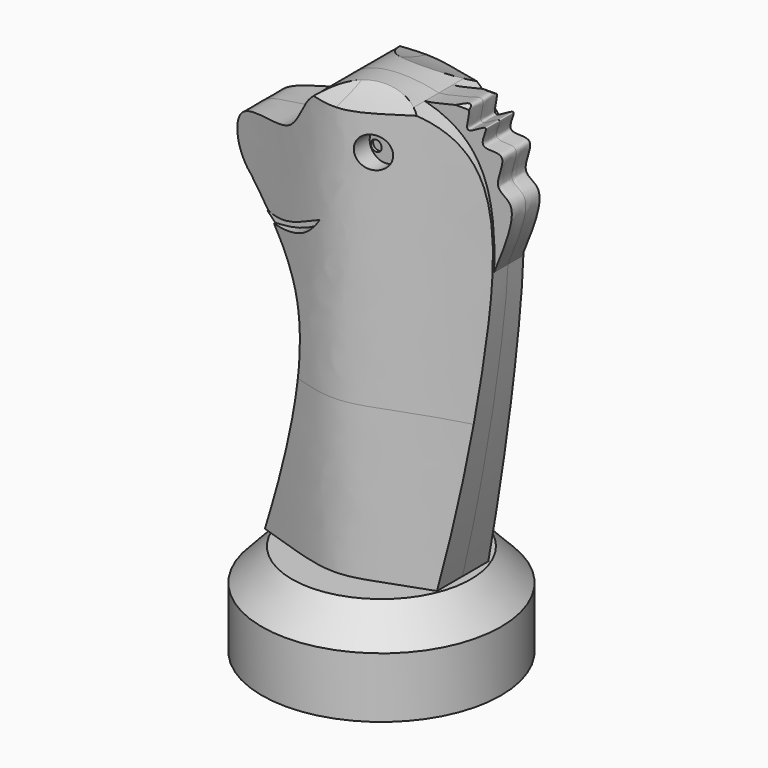
from build123d import *

# Parameters (mm, degrees)
F0_W          = 20.6789579242
F0_H          = 10.4437781447
F0_R          = 2.6884079682
F2_DEPTH      = 10
F3_W          = 121.8075603247
F3_H          = 71.3848918676
F4_DEPTH      = 100
F5_DEPTH      = 3
F6_DEPTH      = 6.25
F8_DEPTH      = 24.9373958048
F8_DEPTH_BACK = 21.754726683
F0_R_2        = 0.9375077203
F9_DEPTH      = 6
F10_DEPTH     = 5.5


# Not quite as in the source:
# - a feature names something its author has since deleted; it is built from what else it names


with BuildPart() as f1:
    # F0 (on Front) → F1 (revolve)
    with BuildSketch(Plane.XZ):
        with Locations((-10.3394789621, -37.1819616321)):
            Rectangle(F0_W, F0_H)
        Polygon((0, -26.4121625388), (-15.4678484998, -26.4121625388), (-20.6789579242, -31.9600725597), (0, -31.9600725597), align=None)
    revolve(axis=Axis((0, 0, -34.4080066216), (0, 0, -1)))


with BuildPart() as f2:
    # F0 (on Front) → F2 (new body, symmetric)
    with BuildSketch(Plane.XZ):
        with BuildLine():
            add(Edge.make_bspline(
                [(-15.4678484998, -26.4121625388), (-13.4170434353, -20.8898176965), (-9.1540550175, -9.4105735163), (-5.5148490257, 10.6849229295), (-11.0633455033, 18.5524195697), (-13.3293069902, 21.0037636867)],
                knots=[0, 0, 0, 0, 0.3292047642, 0.6843147216, 0.8672500498, 0.8672500498, 0.8672500498, 0.8672500498], degree=3))
            Line((-15.4678484998, -26.4121625388), (0, -26.4121625388))
            Line((0, -26.4121625388), (14.038357413, -26.4121625388))
            add(Edge.make_bspline(
                [(21.8767260305, 23.5995116301), (21.7349851157, 19.8558393451), (20.1317592529, 4.274297015), (17.1109510266, -12.943352962), (14.038357413, -26.4121625388)],
                knots=[0.7007538148, 0.7007538148, 0.7007538148, 0.7007538148, 0.7783387637, 1, 1, 1, 1], degree=3))
            add(Edge.make_bspline(
                [(9.9011365003, 45.7942652637), (10.7081780053, 45.5868328827), (16.2676579876, 43.8387084931), (21.4633089561, 38.067196049), (22.0563906808, 28.3448286234), (21.8767260305, 23.5995116301)],
                knots=[0.4564038965, 0.4564038965, 0.4564038965, 0.4564038965, 0.4768115173, 0.6024104908, 0.7007538148, 0.7007538148, 0.7007538148, 0.7007538148], degree=3))
            add(Edge.make_bspline(
                [(-18.6619553715, 26.1048395187), (-21.7267889529, 28.093546629), (-23.7039198678, 37.4882019808), (-7.82054506, 34.9822645389), (-6.2338350146, 46.8698750874), (5.0230557503, 47.0480693103), (9.9011365003, 45.7942652637)],
                knots=[0, 0, 0, 0, 0.1046566415, 0.2239501228, 0.3330520966, 0.4564038965, 0.4564038965, 0.4564038965, 0.4564038965], degree=3))
            add(Edge.make_bspline(
                [(-14.7062902058, 22.4264671244), (-15.9732375567, 23.6830009645), (-17.3175964641, 24.8939202416), (-18.6619553715, 26.1048395187)],
                knots=[0.9032276396, 0.9032276396, 0.9032276396, 0.9032276396, 1, 1, 1, 1], degree=3))
            add(Edge.make_bspline(
                [(-2.9793693684, 26.1795632541), (-6.8807932548, 24.3882648647), (-10.7187069952, 21.6644257307), (-14.7062902058, 22.4264671244)],
                knots=[0, 0, 0, 0, 12.3128551882, 12.3128551882, 12.3128551882, 12.3128551882], degree=3))
            add(Edge.make_bspline(
                [(-13.3293069902, 21.0037636867), (-7.9735843465, 21.242197603), (-5.2197496407, 22.9267347604), (-2.9793693684, 26.1795632541)],
                knots=[0, 0, 0, 0, 11.5719535921, 11.5719535921, 11.5719535921, 11.5719535921], degree=3))
        make_face()
        with Locations((5.4572098888, 38.8016588986)):
            Circle(F0_R, mode=Mode.SUBTRACT)
    extrude(amount=F2_DEPTH, both=True)

    # F3 (on Top) → F4 (cut, symmetric)
    with BuildSketch(Plane.XY):
        Rectangle(F3_W, F3_H)
        with BuildLine():
            add(Edge.make_bspline(
                [(41.3579158485, 0), (12.6386648044, 3.2513821498), (1.5255094939, 15.7927152568), (-14.8981366325, 4.4161337542), (-38.9160625637, 0)],
                knots=[0, 0, 0, 0, 0.5071763346, 1, 1, 1, 1], degree=3))
            add(Edge.make_bspline(
                [(41.3579158485, 0), (12.6386648044, -3.2513821498), (1.5255094939, -15.7927152568), (-14.8981366325, -4.4161337542), (-38.9160625637, 0)],
                knots=[0, 0, 0, 0, 0.5071763346, 1, 1, 1, 1], degree=3))
        make_face(mode=Mode.SUBTRACT)
    extrude(amount=F4_DEPTH, both=True, mode=Mode.SUBTRACT)

    # F0 (on Front) → F5 (join, symmetric)
    with BuildSketch(Plane.XZ):
        with BuildLine():
            add(Edge.make_bspline(
                [(9.9011365003, 45.7942652637), (10.7081780053, 45.5868328827), (16.2676579876, 43.8387084931), (21.4633089561, 38.067196049), (22.0563906808, 28.3448286234), (21.8767260305, 23.5995116301)],
                knots=[0.4564038965, 0.4564038965, 0.4564038965, 0.4564038965, 0.4768115173, 0.6024104908, 0.7007538148, 0.7007538148, 0.7007538148, 0.7007538148], degree=3))
            add(Edge.make_bspline(
                [(9.9011365003, 45.7942652637), (11.1698529182, 45.8964472829), (13.3765379769, 46.5306915245), (15.1636647397, 46.799002489), (18.6143232688, 48.2115693206), (15.8316184726, 41.8456755202), (21.9319277658, 46.8415562154), (18.4163846989, 41.108331158), (25.0756690509, 42.9422779247), (21.1086185991, 36.2564020884), (26.7112040179, 35.3526564288), (23.7214170009, 28.1631973151), (21.8767260305, 23.5995116301)],
                knots=[0, 0, 0, 0, 0.0978972524, 0.1746580424, 0.2503306279, 0.3448082507, 0.4390905105, 0.5250546073, 0.619033764, 0.7311464977, 0.8223963236, 1, 1, 1, 1], degree=3))
        make_face()
    extrude(amount=F5_DEPTH, both=True)

    # F0 (on Front) → F6 (join, symmetric)
    with BuildSketch(Plane.XZ):
        with BuildLine():
            add(Edge.make_bspline(
                [(-13.3293069902, 21.0037636867), (-13.7749499048, 21.4858654979), (-14.2352702587, 21.9593186652), (-14.7062902058, 22.4264671244)],
                knots=[0.8672500498, 0.8672500498, 0.8672500498, 0.8672500498, 0.9032276396, 0.9032276396, 0.9032276396, 0.9032276396], degree=3))
            add(Edge.make_bspline(
                [(-13.3293069902, 21.0037636867), (-7.9735843465, 21.242197603), (-5.2197496407, 22.9267347604), (-2.9793693684, 26.1795632541)],
                knots=[0, 0, 0, 0, 11.5719535921, 11.5719535921, 11.5719535921, 11.5719535921], degree=3))
            add(Edge.make_bspline(
                [(-2.9793693684, 26.1795632541), (-6.8807932548, 24.3882648647), (-10.7187069952, 21.6644257307), (-14.7062902058, 22.4264671244)],
                knots=[0, 0, 0, 0, 12.3128551882, 12.3128551882, 12.3128551882, 12.3128551882], degree=3))
        make_face()
    extrude(amount=F6_DEPTH, both=True)

    # F7 (on Right) → F8 (cut, two sides)
    with BuildSketch(Plane.YZ) as f8_sk:
        with BuildLine():
            add(Edge.make_bspline(
                [(0, 49.1472668946), (-9.6312966198, 39.0917286277), (-42.4910075963, 48.1199361384), (-19.2511547357, 16.8076790869)],
                knots=[0, 0, 0, 0, 37.6358326363, 37.6358326363, 37.6358326363, 37.6358326363], degree=3))
            add(Edge.make_bspline(
                [(0, 49.1472668946), (9.6312966198, 39.0917286277), (42.4910075963, 48.1199361384), (19.2511547357, 16.8076790869)],
                knots=[0, 0, 0, 0, 37.6358326363, 37.6358326363, 37.6358326363, 37.6358326363], degree=3))
            Line((19.2511547357, 16.8076790869), (28.6435540766, 14.3646663055))
            Line((28.6435540766, 14.3646663055), (28.6435540766, 66.1282911897))
            Line((28.6435540766, 66.1282911897), (-29.56193313, 66.1282911897))
            Line((-29.56193313, 66.1282911897), (-29.56193313, 16.8076790869))
            Line((-29.56193313, 16.8076790869), (-19.2511547357, 16.8076790869))
        make_face()
    extrude(amount=F8_DEPTH, mode=Mode.SUBTRACT)
    extrude(f8_sk.sketch, amount=-F8_DEPTH_BACK, mode=Mode.SUBTRACT)

    # F0 (on Front) → F9 (join, symmetric)
    with BuildSketch(Plane.XZ):
        with Locations((5.4572098888, 38.8016588986)):
            Circle(F0_R)
        with Locations((3.9000755642, 38.2443927228)):
            Circle(F0_R_2, mode=Mode.SUBTRACT)
    extrude(amount=F9_DEPTH, both=True)

    # F0 (on Front) → F10 (join, symmetric)
    with BuildSketch(Plane.XZ):
        with Locations((3.9000755642, 38.2443927228)):
            Circle(F0_R_2)
    extrude(amount=F10_DEPTH, both=True)


solid = Compound([f1.part, f2.part])
